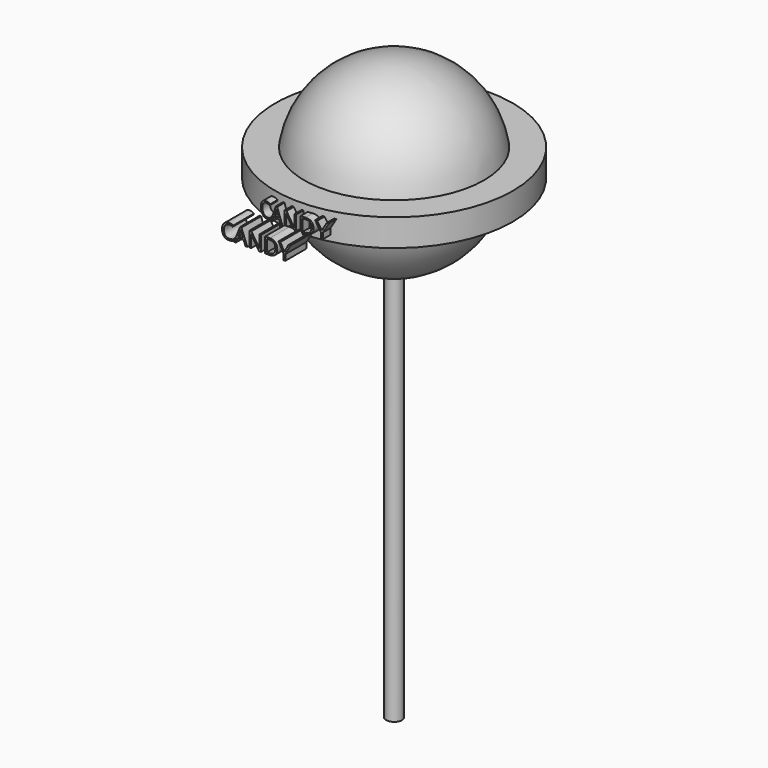
from build123d import *

# Parameters (mm, degrees)
F2_TEXT_SIZE = 3.4899657799
F3_DEPTH     = 28.5


# Not quite as in the source:
# - Text() gives the source's letters only with a copy of the font that has no kerning and outlines rounded to 1/6400 em; it was checked with that copy


with BuildPart() as f1:
    # F0 (on Front) → F1 (revolve)
    with BuildSketch(Plane.XZ):
        with BuildLine():
            Line((0, -12.3562645167), (0, -15.1093733296))
            ThreePointArc((0, -15.1093733296), (0.6571021358, -15.0950779791), (1.3129608706, -15.0522189781))
            Line((1.3129608706, -15.0522189781), (1.3129608706, -12.3562645167))
            Line((1.3129608706, -12.3562645167), (0, -12.3562645167))
        make_face()
        with BuildLine():
            ThreePointArc((1.3129608706, -15.0522189781), (0.6571021358, -15.0950779791), (0, -15.1093733296))
            Line((0, -15.1093733296), (0, -81.0881704092))
            Line((0, -81.0881704092), (1.3129608706, -81.0881704092))
            Line((1.3129608706, -81.0881704092), (1.3129608706, -15.0522189781))
        make_face()
        with BuildLine():
            Line((1.3129608706, -12.3562645167), (1.3129608706, -15.0522189781))
            ThreePointArc((1.3129608706, -15.0522189781), (10.3439191265, -11.0134690047), (14.9404197859, -2.2532241419))
            Line((14.9404197859, -2.2532241419), (5.7882774271, -2.2532241419))
            Line((5.7882774271, -2.2532241419), (5.7882774271, 2.2532241419))
            Line((5.7882774271, 2.2532241419), (14.9404197859, 2.2532241419))
            ThreePointArc((14.9404197859, 2.2532241419), (9.8551600103, 11.4529028453), (0, 15.1093733296))
            Line((0, 15.1093733296), (0, -12.3562645167))
            Line((0, -12.3562645167), (1.3129608706, -12.3562645167))
        make_face()
        with BuildLine():
            Line((5.7882774271, -2.2532241419), (14.9404197859, -2.2532241419))
            ThreePointArc((14.9404197859, -2.2532241419), (15.1093733296, 0), (14.9404197859, 2.2532241419))
            Line((14.9404197859, 2.2532241419), (5.7882774271, 2.2532241419))
            Line((5.7882774271, 2.2532241419), (5.7882774271, -2.2532241419))
        make_face()
        with BuildLine():
            ThreePointArc((14.9404197859, 2.2532241419), (15.1093733296, 0), (14.9404197859, -2.2532241419))
            Line((14.9404197859, -2.2532241419), (19.7244663142, -2.2532241419))
            Line((19.7244663142, -2.2532241419), (19.7244663142, 2.2532241419))
            Line((19.7244663142, 2.2532241419), (14.9404197859, 2.2532241419))
        make_face()
    revolve(axis=Axis((0, 0, 17.9043356329), (0, 0, 1)))

    # F2 (on Front) → F3 (join)
    with BuildSketch(Plane.XZ):
        with Locations((-5.9742112644, -1.2590244878)):
            Text('CANDY', F2_TEXT_SIZE, font='Open Sans', text_align=(TextAlign.LEFT, TextAlign.BOTTOM))
    extrude(amount=F3_DEPTH)

    # F4 (on Front) → F6 (revolve, cut)
    with BuildSketch(Plane.XZ):
        Polygon((21.2244663142, 3.7532241419), (21.2244663142, -3.7532241419), (14.8748876527, -3.7532241419), (24.5479121804, -7.6714825213), (24.5479121804, 9.5449505702), (13.7858726084, 9.5449505702), (15.5795449391, 3.7532241419), align=None)
    revolve(axis=Axis((0, 0, 22.4731564522), (0, 0, 1)), mode=Mode.SUBTRACT)


solid = f1.part
